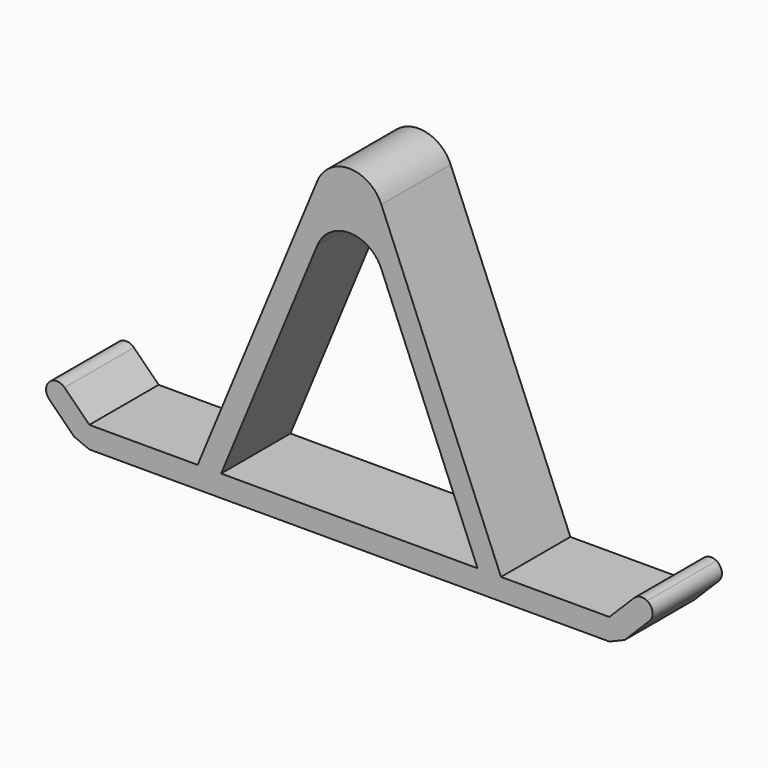
from build123d import *

# Parameters (mm, degrees)
F1_DEPTH = 20
F2_R     = 8
F3_R     = 2.49999


# Not quite as in the source:
# - a fillet or chamfer is up to 0.001 mm smaller than in the source, because OpenCascade refuses the exact size


with BuildPart() as f1:
    # F0 (on Front) → F1 (new body)
    with BuildSketch(Plane.XZ):
        Polygon((-35, 0), (-29.5880389985, 0), (0, 71.4318450343), (0, 84.4974746831), align=None)
        Polygon((0, 71.4318450343), (29.5880389985, 0), (35, 0), (0, 84.4974746831), align=None)
        Polygon((0, -5), (0, 0), (-29.5880389985, 0), (-35, 0), (-60, 0), (-67.0710678119, 7.0710678119), (-71.5539451727, 4.4828773608), (-63.5355339059, -3.5355339059), (-60, -5), align=None)
        Polygon((29.5880389985, 0), (0, 0), (0, -5), (60, -5), (63.5355339059, -3.5355339059), (71.5539451727, 4.4828773608), (67.0710678119, 7.0710678119), (60, 0), (35, 0), align=None)
    extrude(amount=F1_DEPTH)

    # F2
    f2_edges = [f1.edges().sort_by_distance(p)[0] for p in [
        (0, -10, 84.497475),
        (0, -10, 71.431845),
    ]]
    fillet(f2_edges, radius=F2_R)

    # F3 (radius 2.5 in the source; OpenCascade refuses exactly that, so slightly less here)
    f3_edges = [f1.edges().sort_by_distance(p)[0] for p in [
        (-67.071068, -10, 7.071068),
        (-71.553945, -10, 4.482877),
        (67.071068, -10, 7.071068),
        (71.553945, -10, 4.482877),
    ]]
    fillet(f3_edges, radius=F3_R)


solid = f1.part
